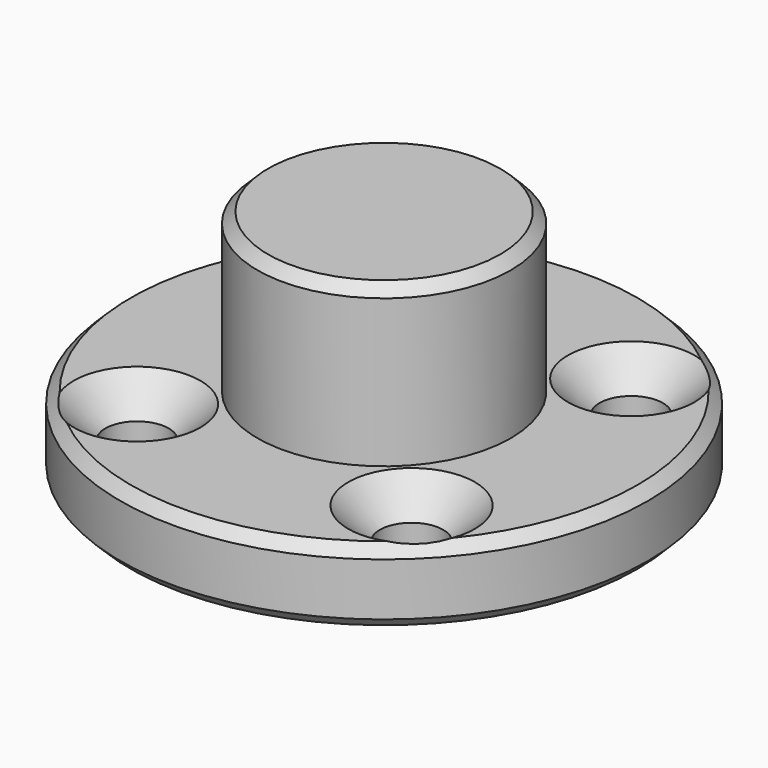
from build123d import *

# Parameters (mm, degrees)
F0_R     = 25
F0_R_2   = 3
F1_DEPTH = 7
F2_R     = 12
F3_DEPTH = 15
F4_SIZE  = 1


# Not quite as in the source:
# - a fillet or chamfer that OpenCascade refuses, or shapes differently, is made with other operations: its cross-section is extruded or revolved along the edge and cut away or added


with BuildPart() as f1:
    # F0 (on Top) → F1 (new body)
    with BuildSketch(Plane.XY):
        Circle(F0_R)
        with Locations((-13, -13)):
            Circle(F0_R_2, mode=Mode.SUBTRACT)
        with Locations((13, -13)):
            Circle(F0_R_2, mode=Mode.SUBTRACT)
        with Locations((-13, 13)):
            Circle(F0_R_2, mode=Mode.SUBTRACT)
        with Locations((13, 13)):
            Circle(F0_R_2, mode=Mode.SUBTRACT)
    extrude(amount=F1_DEPTH)

    # F2 (on face) → F3 (join)
    with BuildSketch(Plane.XY.offset(7)):
        Circle(F2_R)
    extrude(amount=F3_DEPTH)

    # F4
    f4_edges = [f1.edges().sort_by_distance(p)[0] for p in [
        (-12, 0, 22),
        (-25, 0, 7),
        (-25, 0, 0),
    ]]
    chamfer(f4_edges, length=F4_SIZE)

    # F5: chamfer of 3 on 4 edges, made by hand

    # F5_s1 → F5_t2 (revolve, cut)
    with BuildSketch(Plane.XZ.offset(13)):
        Polygon((-7, 7), (-10, 4), (-10, 7), align=None)
    revolve(axis=Axis((-13, -13, 7), (0, 0, 1)), mode=Mode.SUBTRACT)

    # F5_s3 → F5_t4 (revolve, cut)
    with BuildSketch(Plane.XZ.offset(13)):
        Polygon((19, 7), (16, 4), (16, 7), align=None)
    revolve(axis=Axis((13, -13, 7), (0, 0, 1)), mode=Mode.SUBTRACT)

    # F5_s5 → F5_t6 (revolve, cut)
    with BuildSketch(Plane.XZ.offset(-13)):
        Polygon((19, 7), (16, 4), (16, 7), align=None)
    revolve(axis=Axis((13, 13, 7), (0, 0, 1)), mode=Mode.SUBTRACT)

    # F5_s7 → F5_t8 (revolve, cut)
    with BuildSketch(Plane.XZ.offset(-13)):
        Polygon((-7, 7), (-10, 4), (-10, 7), align=None)
    revolve(axis=Axis((-13, 13, 7), (0, 0, 1)), mode=Mode.SUBTRACT)


solid = f1.part
